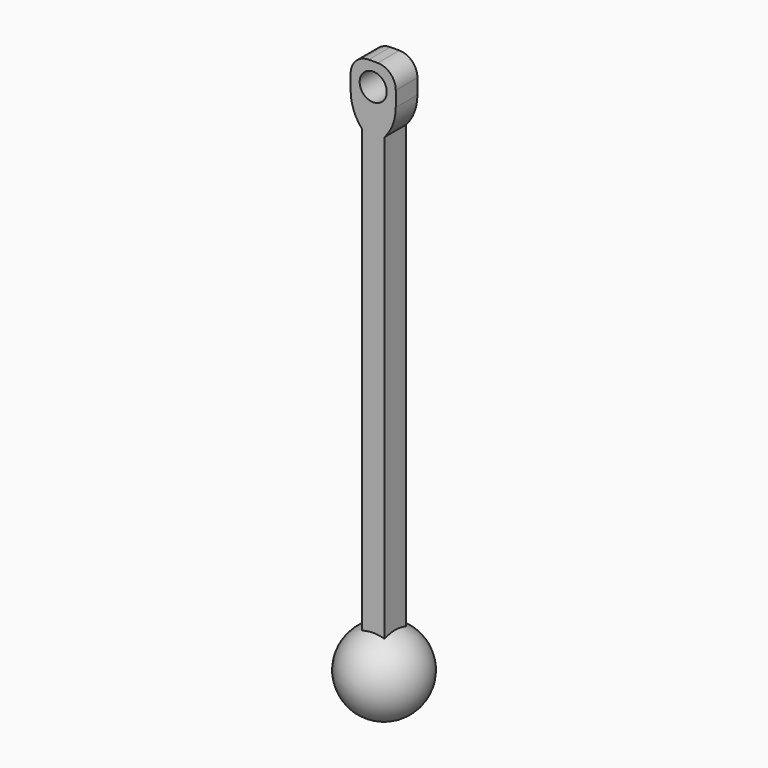
from build123d import *

# Parameters (mm, degrees)
F0_R        = 1.5
F1_DEPTH    = 3
F2_R        = 2
F3_R        = 2
F4_T1_DEPTH = 19.5359456942


# Not quite as in the source:
# - a fillet or chamfer that OpenCascade refuses, or shapes differently, is made with other operations: its cross-section is extruded or revolved along the edge and cut away or added


with BuildPart() as f1:
    # F0 (on Front) → F1 (new body)
    with BuildSketch(Plane.XZ):
        Polygon((-14.9506077915, 50.13686046), (-19.9506077915, 50.13686046), (-19.9506077915, 43.13686046), (-18.7006077915, 43.13686046), (-18.7006077915, 10.13686046), (-18.7006077915, -9.86313954), (-17.4506077915, -9.86313954), (-16.2006077915, -9.86313954), (-16.2006077915, 10.13686046), (-16.2006077915, 43.13686046), (-14.9506077915, 43.13686046), align=None)
        with Locations((-17.4506077915, 47.63686046)):
            Circle(F0_R, mode=Mode.SUBTRACT)
    extrude(amount=F1_DEPTH)

    # F2
    f2_edges = [f1.edges().sort_by_distance(p)[0] for p in [
        (-14.950608, -1.5, 50.13686),
    ]]
    fillet(f2_edges, radius=F2_R)

    # F3
    f3_edges = [f1.edges().sort_by_distance(p)[0] for p in [
        (-19.950608, -1.5, 50.13686),
    ]]
    fillet(f3_edges, radius=F3_R)

    # F4: fillet of radius 5 on 2 edges, made by hand

    # F4_s2 → F4_t1 (cut)
    with BuildSketch(Plane.XZ.offset(-8.2679728471)):
        with BuildLine():
            ThreePointArc((-14.9506077915, 46.4440495989), (-15.2735360581, 44.6762826459), (-16.2006077915, 43.13686046))
            Line((-16.2006077915, 43.13686046), (-14.9506077915, 43.13686046))
            Line((-14.9506077915, 43.13686046), (-14.9506077915, 46.4440495989))
        make_face()
        with BuildLine():
            ThreePointArc((-19.9506077915, 46.4440495989), (-19.627679525, 44.6762826459), (-18.7006077915, 43.13686046))
            Line((-18.7006077915, 43.13686046), (-19.9506077915, 43.13686046))
            Line((-19.9506077915, 43.13686046), (-19.9506077915, 46.4440495989))
        make_face()
    extrude(amount=F4_T1_DEPTH, mode=Mode.SUBTRACT)

    # F5 (on face) → F6 (revolve)
    with BuildSketch(Plane(origin=(0, 0, -9.86313954), x_dir=(1, 0, 0), z_dir=(0, 0, -1))):
        with BuildLine():
            Line((-17.4506077915, 3), (-17.4506077915, 6))
            ThreePointArc((-17.4506077915, 6), (-21.9506077915, 1.5), (-17.4506077915, -3))
            Line((-17.4506077915, -3), (-17.4506077915, 0))
            Line((-17.4506077915, 0), (-18.7006077915, 0))
            Line((-18.7006077915, 0), (-18.7006077915, 3))
            Line((-18.7006077915, 3), (-17.4506077915, 3))
        make_face()
    revolve(axis=Axis((-17.4506077915, -1.5, -9.86313954), (0, 1, 0)))


solid = f1.part
